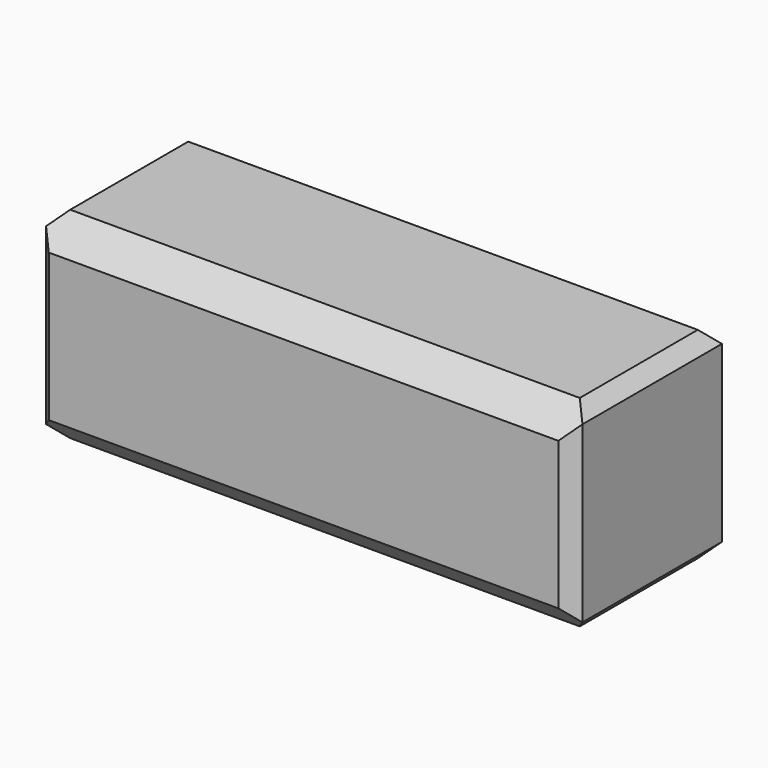
from build123d import *

# Parameters (mm, degrees)
F0_W     = 203.2
F0_H     = 76.2
F1_DEPTH = 76.2
F2_SIZE  = 10.16
F3_SIZE  = 5.07999
F4_R     = 12.7
F5_DEPTH = 50.8


# Not quite as in the source:
# - a fillet or chamfer is up to 0.001 mm smaller than in the source, because OpenCascade refuses the exact size


with BuildPart() as f1:
    # F0 (on Front) → F1 (new body)
    with BuildSketch(Plane.XZ):
        with Locations((4.1285920888, -9.8249100385)):
            Rectangle(F0_W, F0_H)
    extrude(amount=F1_DEPTH)

    # F2
    f2_edges = [f1.edges().sort_by_distance(p)[0] for p in [
        (4.128592, -76.2, 28.27509),
        (4.128592, -76.2, -47.92491),
        (4.128592, 0, 28.27509),
        (4.128592, 0, -47.92491),
    ]]
    chamfer(f2_edges, length=F2_SIZE)

    # F3 (size 5.08 in the source; OpenCascade refuses exactly that, so slightly less here)
    f3_edges = [f1.edges().sort_by_distance(p)[0] for p in [
        (-97.471408, -38.1, 28.27509),
        (-97.471408, -76.2, -9.82491),
        (-97.471408, -38.1, -47.92491),
        (-97.471408, 0, -9.82491),
        (105.728592, 0, -9.82491),
        (105.728592, -38.1, -47.92491),
        (105.728592, -76.2, -9.82491),
        (105.728592, -38.1, 28.27509),
    ]]
    chamfer(f3_edges, length=F3_SIZE)

    # F4 (on face) → F5 (cut)
    with BuildSketch(Plane(origin=(0, 0, -47.9249100385), x_dir=(1, 0, 0), z_dir=(0, 0, -1))):
        with Locations((0, 38.1)):
            Circle(F4_R)
    extrude(amount=-F5_DEPTH, mode=Mode.SUBTRACT)


solid = f1.part
